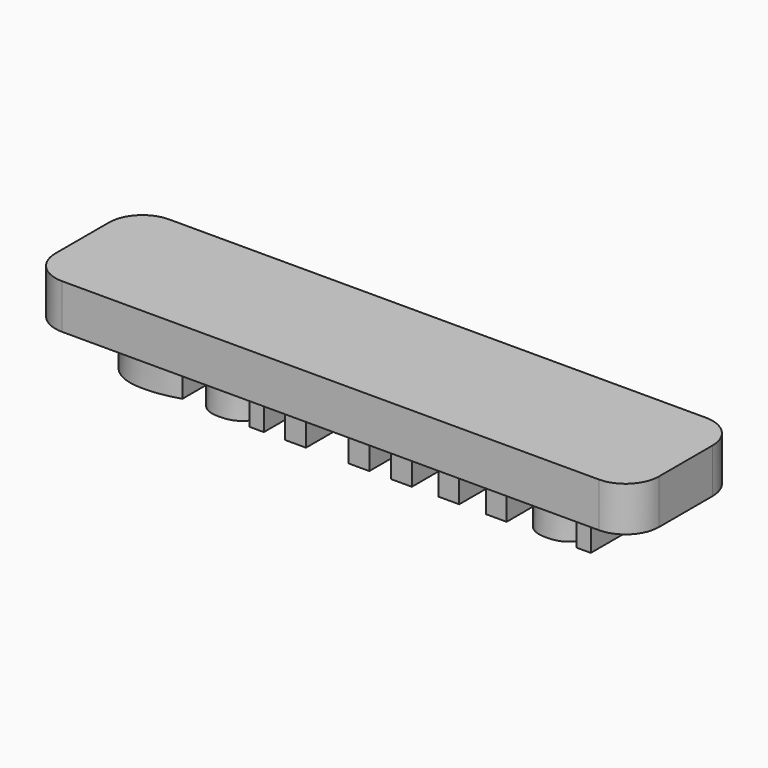
from build123d import *

# Parameters (mm, degrees)
F1_W         = 54.1251940079
F1_H         = 12
F2_DEPTH     = 4
F0_TEXT_SIZE = 12.5
F3_DEPTH     = 3
F4_R         = 3


# Not quite as in the source:
# - Text() gives the source's letters only with a copy of the font that has no kerning and outlines rounded to 1/6400 em; it was checked with that copy


with BuildPart() as f2:
    # F1 (on Top) → F2 (new body)
    with BuildSketch(Plane.XY):
        with Locations((-0.0989846885, 0.0495596323)):
            Rectangle(F1_W, F1_H)
    extrude(amount=F2_DEPTH)

    # F0 (on Top) → F3 (join)
    with BuildSketch(Plane.XY):
        with Locations((-22.892578125, -4.5)):
            Text('Garima', F0_TEXT_SIZE, font='Open Sans', font_style=FontStyle.BOLD, text_align=(TextAlign.LEFT, TextAlign.BOTTOM))
    extrude(amount=-F3_DEPTH)

    # F4
    f4_edges = [f2.edges().sort_by_distance(p)[0] for p in [
        (-27.161582, 6.04956, 2),
        (26.963612, 6.04956, 2),
        (26.963612, -5.95044, 2),
        (-27.161582, -5.95044, 2),
    ]]
    fillet(f4_edges, radius=F4_R)


solid = f2.part
